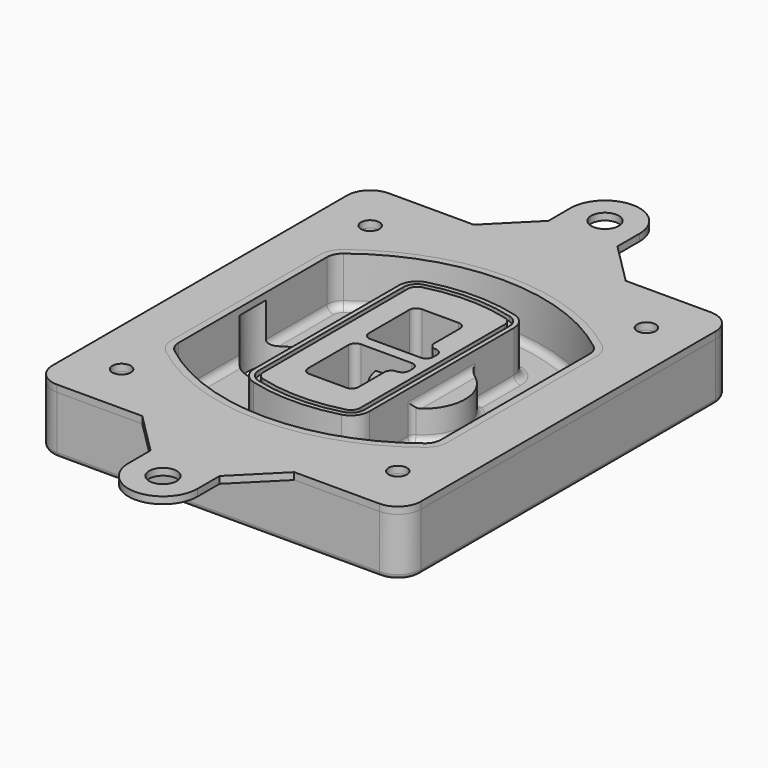
from build123d import *

# Parameters (mm, degrees)
F0_R      = 4
F1_DEPTH  = 25
F2_DEPTH  = 3
F3_DEPTH  = 18
F5_DEPTH  = 21
F6_DEPTH  = 2
F8_DEPTH  = 20
F9_DEPTH  = 16
F10_DEPTH = 25
F7_R      = 6
F7_R_2    = 4
F11_DEPTH = 6
F13_DEPTH = 9
F14_R     = 3
F15_R     = 2
F16_R     = 6
F16_R_2   = 4
F17_DEPTH = 3


with BuildPart() as f1:
    # F0 (on Top) → F1 (new body)
    with BuildSketch(Plane.XY):
        with BuildLine():
            ThreePointArc((-80, -80), (-77.0710678119, -87.0710678119), (-70, -90))
            Line((-70, -90), (70, -90))
            ThreePointArc((70, -90), (77.0710678119, -87.0710678119), (80, -80))
            Line((80, -80), (80, 80))
            ThreePointArc((80, 80), (77.0710678119, 87.0710678119), (70, 90))
            Line((70, 90), (-70, 90))
            ThreePointArc((-70, 90), (-77.0710678119, 87.0710678119), (-80, 80))
            Line((-80, 80), (-80, -80))
        make_face()
        with Locations((-60, -67.5)):
            Circle(F0_R, mode=Mode.SUBTRACT)
        with Locations((60, -67.5)):
            Circle(F0_R, mode=Mode.SUBTRACT)
        with Locations((-60, 67.5)):
            Circle(F0_R, mode=Mode.SUBTRACT)
        with BuildLine():
            ThreePointArc((-64, 40.2934422872), (-62.5820384798, 46.4328484224), (-58.6153846154, 51.3286200352))
            ThreePointArc((-58.6153846154, 51.3286200352), (0, 71.5), (58.6153846154, 51.3286200352))
            ThreePointArc((58.6153846154, 51.3286200352), (62.5820384798, 46.4328484224), (64, 40.2934422872))
            Line((64, 40.2934422872), (64, -40.2934422872))
            ThreePointArc((64, -40.2934422872), (62.5820384798, -46.4328484224), (58.6153846154, -51.3286200352))
            ThreePointArc((58.6153846154, -51.3286200352), (0, -71.5), (-58.6153846154, -51.3286200352))
            ThreePointArc((-58.6153846154, -51.3286200352), (-62.5820384798, -46.4328484224), (-64, -40.2934422872))
            Line((-64, -40.2934422872), (-64, 40.2934422872))
        make_face(mode=Mode.SUBTRACT)
        with Locations((60, 67.5)):
            Circle(F0_R, mode=Mode.SUBTRACT)
        with BuildLine():
            ThreePointArc((58.6153846154, 51.3286200352), (0, 71.5), (-58.6153846154, 51.3286200352))
            ThreePointArc((-58.6153846154, 51.3286200352), (-62.5820384798, 46.4328484224), (-64, 40.2934422872))
            Line((-64, 40.2934422872), (-64, -40.2934422872))
            ThreePointArc((-64, -40.2934422872), (-62.5820384798, -46.4328484224), (-58.6153846154, -51.3286200352))
            ThreePointArc((-58.6153846154, -51.3286200352), (0, -71.5), (58.6153846154, -51.3286200352))
            ThreePointArc((58.6153846154, -51.3286200352), (62.5820384798, -46.4328484224), (64, -40.2934422872))
            Line((64, -40.2934422872), (64, 40.2934422872))
            ThreePointArc((64, 40.2934422872), (62.5820384798, 46.4328484224), (58.6153846154, 51.3286200352))
        make_face()
        with BuildLine():
            Line((-60, -40.2934422872), (-60, 40.2934422872))
            ThreePointArc((-60, 40.2934422872), (-58.9871703427, 44.6787323838), (-56.1538461538, 48.1757121072))
            ThreePointArc((-56.1538461538, 48.1757121072), (0, 67.5), (56.1538461538, 48.1757121072))
            ThreePointArc((56.1538461538, 48.1757121072), (58.9871703427, 44.6787323838), (60, 40.2934422872))
            Line((60, 40.2934422872), (60, -40.2934422872))
            ThreePointArc((60, -40.2934422872), (58.9871703427, -44.6787323838), (56.1538461538, -48.1757121072))
            ThreePointArc((56.1538461538, -48.1757121072), (0, -67.5), (-56.1538461538, -48.1757121072))
            ThreePointArc((-56.1538461538, -48.1757121072), (-58.9871703427, -44.6787323838), (-60, -40.2934422872))
        make_face(mode=Mode.SUBTRACT)
        with BuildLine():
            ThreePointArc((-56.1538461538, 48.1757121072), (-58.9871703427, 44.6787323838), (-60, 40.2934422872))
            Line((-60, 40.2934422872), (-60, -40.2934422872))
            ThreePointArc((-60, -40.2934422872), (-58.9871703427, -44.6787323838), (-56.1538461538, -48.1757121072))
            ThreePointArc((-56.1538461538, -48.1757121072), (0, -67.5), (56.1538461538, -48.1757121072))
            ThreePointArc((56.1538461538, -48.1757121072), (58.9871703427, -44.6787323838), (60, -40.2934422872))
            Line((60, -40.2934422872), (60, 40.2934422872))
            ThreePointArc((60, 40.2934422872), (58.9871703427, 44.6787323838), (56.1538461538, 48.1757121072))
            ThreePointArc((56.1538461538, 48.1757121072), (0, 67.5), (-56.1538461538, 48.1757121072))
        make_face()
        with BuildLine():
            ThreePointArc((54.3076923077, 45.8110311612), (56.2910192399, 43.3631453548), (57, 40.2934422872))
            Line((57, 40.2934422872), (57, -40.2934422872))
            ThreePointArc((57, -40.2934422872), (56.2910192399, -43.3631453548), (54.3076923077, -45.8110311612))
            ThreePointArc((54.3076923077, -45.8110311612), (0, -64.5), (-54.3076923077, -45.8110311612))
            ThreePointArc((-54.3076923077, -45.8110311612), (-56.2910192399, -43.3631453548), (-57, -40.2934422872))
            Line((-57, -40.2934422872), (-57, 40.2934422872))
            ThreePointArc((-57, 40.2934422872), (-56.2910192399, 43.3631453548), (-54.3076923077, 45.8110311612))
            ThreePointArc((-54.3076923077, 45.8110311612), (0, 64.5), (54.3076923077, 45.8110311612))
        make_face(mode=Mode.SUBTRACT)
        with BuildLine():
            Line((57, -40.2934422872), (57, 40.2934422872))
            ThreePointArc((57, 40.2934422872), (56.2910192399, 43.3631453548), (54.3076923077, 45.8110311612))
            ThreePointArc((54.3076923077, 45.8110311612), (0, 64.5), (-54.3076923077, 45.8110311612))
            ThreePointArc((-54.3076923077, 45.8110311612), (-56.2910192399, 43.3631453548), (-57, 40.2934422872))
            Line((-57, 40.2934422872), (-57, -40.2934422872))
            ThreePointArc((-57, -40.2934422872), (-56.2910192399, -43.3631453548), (-54.3076923077, -45.8110311612))
            ThreePointArc((-54.3076923077, -45.8110311612), (0, -64.5), (54.3076923077, -45.8110311612))
            ThreePointArc((54.3076923077, -45.8110311612), (56.2910192399, -43.3631453548), (57, -40.2934422872))
        make_face()
    extrude(amount=-F1_DEPTH)

    # F0 (on Top) → F2 (join)
    with BuildSketch(Plane.XY):
        with BuildLine():
            ThreePointArc((-56.1538461538, 48.1757121072), (-58.9871703427, 44.6787323838), (-60, 40.2934422872))
            Line((-60, 40.2934422872), (-60, -40.2934422872))
            ThreePointArc((-60, -40.2934422872), (-58.9871703427, -44.6787323838), (-56.1538461538, -48.1757121072))
            ThreePointArc((-56.1538461538, -48.1757121072), (0, -67.5), (56.1538461538, -48.1757121072))
            ThreePointArc((56.1538461538, -48.1757121072), (58.9871703427, -44.6787323838), (60, -40.2934422872))
            Line((60, -40.2934422872), (60, 40.2934422872))
            ThreePointArc((60, 40.2934422872), (58.9871703427, 44.6787323838), (56.1538461538, 48.1757121072))
            ThreePointArc((56.1538461538, 48.1757121072), (0, 67.5), (-56.1538461538, 48.1757121072))
        make_face()
        with BuildLine():
            ThreePointArc((54.3076923077, 45.8110311612), (56.2910192399, 43.3631453548), (57, 40.2934422872))
            Line((57, 40.2934422872), (57, -40.2934422872))
            ThreePointArc((57, -40.2934422872), (56.2910192399, -43.3631453548), (54.3076923077, -45.8110311612))
            ThreePointArc((54.3076923077, -45.8110311612), (0, -64.5), (-54.3076923077, -45.8110311612))
            ThreePointArc((-54.3076923077, -45.8110311612), (-56.2910192399, -43.3631453548), (-57, -40.2934422872))
            Line((-57, -40.2934422872), (-57, 40.2934422872))
            ThreePointArc((-57, 40.2934422872), (-56.2910192399, 43.3631453548), (-54.3076923077, 45.8110311612))
            ThreePointArc((-54.3076923077, 45.8110311612), (0, 64.5), (54.3076923077, 45.8110311612))
        make_face(mode=Mode.SUBTRACT)
    extrude(amount=F2_DEPTH)

    # F0 (on Top) → F3 (cut)
    with BuildSketch(Plane.XY):
        with BuildLine():
            Line((57, -40.2934422872), (57, 40.2934422872))
            ThreePointArc((57, 40.2934422872), (56.2910192399, 43.3631453548), (54.3076923077, 45.8110311612))
            ThreePointArc((54.3076923077, 45.8110311612), (0, 64.5), (-54.3076923077, 45.8110311612))
            ThreePointArc((-54.3076923077, 45.8110311612), (-56.2910192399, 43.3631453548), (-57, 40.2934422872))
            Line((-57, 40.2934422872), (-57, -40.2934422872))
            ThreePointArc((-57, -40.2934422872), (-56.2910192399, -43.3631453548), (-54.3076923077, -45.8110311612))
            ThreePointArc((-54.3076923077, -45.8110311612), (0, -64.5), (54.3076923077, -45.8110311612))
            ThreePointArc((54.3076923077, -45.8110311612), (56.2910192399, -43.3631453548), (57, -40.2934422872))
        make_face()
    extrude(amount=-F3_DEPTH, mode=Mode.SUBTRACT)

    # F4 (on face) → F5 (join, through all)
    with BuildSketch(Plane.XY.offset(3)):
        with BuildLine():
            ThreePointArc((-25, -39.2465276821), (-23.3511545998, -44.1109737193), (-19.0842911877, -46.9702398883))
            ThreePointArc((-19.0842911877, -46.9702398883), (0, -49.5), (19.0842911877, -46.9702398883))
            ThreePointArc((19.0842911877, -46.9702398883), (23.3511545998, -44.1109737193), (25, -39.2465276821))
            Line((25, -39.2465276821), (25, 39.2465276821))
            ThreePointArc((25, 39.2465276821), (23.3511545998, 44.1109737193), (19.0842911877, 46.9702398883))
            ThreePointArc((19.0842911877, 46.9702398883), (0, 49.5), (-19.0842911877, 46.9702398883))
            ThreePointArc((-19.0842911877, 46.9702398883), (-23.3511545998, 44.1109737193), (-25, 39.2465276821))
            Line((-25, 39.2465276821), (-25, -39.2465276821))
        make_face()
        with BuildLine():
            ThreePointArc((18.5632183908, 45.0393118368), (21.7633659499, 42.89486221), (23, 39.2465276821))
            Line((23, 39.2465276821), (23, -39.2465276821))
            ThreePointArc((23, -39.2465276821), (21.7633659499, -42.89486221), (18.5632183908, -45.0393118368))
            ThreePointArc((18.5632183908, -45.0393118368), (0, -47.5), (-18.5632183908, -45.0393118368))
            ThreePointArc((-18.5632183908, -45.0393118368), (-21.7633659499, -42.89486221), (-23, -39.2465276821))
            Line((-23, -39.2465276821), (-23, 39.2465276821))
            ThreePointArc((-23, 39.2465276821), (-21.7633659499, 42.89486221), (-18.5632183908, 45.0393118368))
            ThreePointArc((-18.5632183908, 45.0393118368), (0, 47.5), (18.5632183908, 45.0393118368))
        make_face(mode=Mode.SUBTRACT)
        with BuildLine():
            Line((23, -39.2465276821), (23, 39.2465276821))
            ThreePointArc((23, 39.2465276821), (21.7633659499, 42.89486221), (18.5632183908, 45.0393118368))
            ThreePointArc((18.5632183908, 45.0393118368), (0, 47.5), (-18.5632183908, 45.0393118368))
            ThreePointArc((-18.5632183908, 45.0393118368), (-21.7633659499, 42.89486221), (-23, 39.2465276821))
            Line((-23, 39.2465276821), (-23, -39.2465276821))
            ThreePointArc((-23, -39.2465276821), (-21.7633659499, -42.89486221), (-18.5632183908, -45.0393118368))
            ThreePointArc((-18.5632183908, -45.0393118368), (0, -47.5), (18.5632183908, -45.0393118368))
            ThreePointArc((18.5632183908, -45.0393118368), (21.7633659499, -42.89486221), (23, -39.2465276821))
        make_face()
        with BuildLine():
            ThreePointArc((18.0421455939, 43.1083837852), (20.1755772999, 41.6787507007), (21, 39.2465276821))
            Line((21, 39.2465276821), (21, -39.2465276821))
            ThreePointArc((21, -39.2465276821), (20.1755772999, -41.6787507007), (18.0421455939, -43.1083837852))
            ThreePointArc((18.0421455939, -43.1083837852), (0, -45.5), (-18.0421455939, -43.1083837852))
            ThreePointArc((-18.0421455939, -43.1083837852), (-20.1755772999, -41.6787507007), (-21, -39.2465276821))
            Line((-21, -39.2465276821), (-21, 39.2465276821))
            ThreePointArc((-21, 39.2465276821), (-20.1755772999, 41.6787507007), (-18.0421455939, 43.1083837852))
            ThreePointArc((-18.0421455939, 43.1083837852), (0, 45.5), (18.0421455939, 43.1083837852))
        make_face(mode=Mode.SUBTRACT)
        with BuildLine():
            Line((21, -39.2465276821), (21, 39.2465276821))
            ThreePointArc((21, 39.2465276821), (20.1755772999, 41.6787507007), (18.0421455939, 43.1083837852))
            ThreePointArc((18.0421455939, 43.1083837852), (0, 45.5), (-18.0421455939, 43.1083837852))
            ThreePointArc((-18.0421455939, 43.1083837852), (-20.1755772999, 41.6787507007), (-21, 39.2465276821))
            Line((-21, 39.2465276821), (-21, -39.2465276821))
            ThreePointArc((-21, -39.2465276821), (-20.1755772999, -41.6787507007), (-18.0421455939, -43.1083837852))
            ThreePointArc((-18.0421455939, -43.1083837852), (0, -45.5), (18.0421455939, -43.1083837852))
            ThreePointArc((18.0421455939, -43.1083837852), (20.1755772999, -41.6787507007), (21, -39.2465276821))
        make_face()
        with BuildLine():
            Line((-8, -2.5), (14, -2.5))
            ThreePointArc((14, -2.5), (16.1213203436, -3.3786796564), (17, -5.5))
            Line((17, -5.5), (17, -7.5))
            ThreePointArc((17, -7.5), (16.1213203436, -9.6213203436), (14, -10.5))
            ThreePointArc((14, -10.5), (11.8786796564, -11.3786796564), (11, -13.5))
            Line((11, -13.5), (11, -27.5))
            ThreePointArc((11, -27.5), (10.1213203436, -29.6213203436), (8, -30.5))
            Line((8, -30.5), (-8, -30.5))
            ThreePointArc((-8, -30.5), (-10.1213203436, -29.6213203436), (-11, -27.5))
            Line((-11, -27.5), (-11, -5.5))
            ThreePointArc((-11, -5.5), (-10.1213203436, -3.3786796564), (-8, -2.5))
        make_face(mode=Mode.SUBTRACT)
        with BuildLine():
            ThreePointArc((-8, 2.5), (-10.1213203436, 3.3786796564), (-11, 5.5))
            Line((-11, 5.5), (-11, 27.5))
            ThreePointArc((-11, 27.5), (-10.1213203436, 29.6213203436), (-8, 30.5))
            Line((-8, 30.5), (8, 30.5))
            ThreePointArc((8, 30.5), (10.1213203436, 29.6213203436), (11, 27.5))
            Line((11, 27.5), (11, 13.5))
            ThreePointArc((11, 13.5), (11.8786796564, 11.3786796564), (14, 10.5))
            ThreePointArc((14, 10.5), (16.1213203436, 9.6213203436), (17, 7.5))
            Line((17, 7.5), (17, 5.5))
            ThreePointArc((17, 5.5), (16.1213203436, 3.3786796564), (14, 2.5))
            Line((14, 2.5), (-8, 2.5))
        make_face(mode=Mode.SUBTRACT)
    extrude(amount=-F5_DEPTH)

    # F4 (on face) → F6 (cut)
    with BuildSketch(Plane.XY.offset(3)):
        with BuildLine():
            Line((23, -39.2465276821), (23, 39.2465276821))
            ThreePointArc((23, 39.2465276821), (21.7633659499, 42.89486221), (18.5632183908, 45.0393118368))
            ThreePointArc((18.5632183908, 45.0393118368), (0, 47.5), (-18.5632183908, 45.0393118368))
            ThreePointArc((-18.5632183908, 45.0393118368), (-21.7633659499, 42.89486221), (-23, 39.2465276821))
            Line((-23, 39.2465276821), (-23, -39.2465276821))
            ThreePointArc((-23, -39.2465276821), (-21.7633659499, -42.89486221), (-18.5632183908, -45.0393118368))
            ThreePointArc((-18.5632183908, -45.0393118368), (0, -47.5), (18.5632183908, -45.0393118368))
            ThreePointArc((18.5632183908, -45.0393118368), (21.7633659499, -42.89486221), (23, -39.2465276821))
        make_face()
        with BuildLine():
            ThreePointArc((18.0421455939, 43.1083837852), (20.1755772999, 41.6787507007), (21, 39.2465276821))
            Line((21, 39.2465276821), (21, -39.2465276821))
            ThreePointArc((21, -39.2465276821), (20.1755772999, -41.6787507007), (18.0421455939, -43.1083837852))
            ThreePointArc((18.0421455939, -43.1083837852), (0, -45.5), (-18.0421455939, -43.1083837852))
            ThreePointArc((-18.0421455939, -43.1083837852), (-20.1755772999, -41.6787507007), (-21, -39.2465276821))
            Line((-21, -39.2465276821), (-21, 39.2465276821))
            ThreePointArc((-21, 39.2465276821), (-20.1755772999, 41.6787507007), (-18.0421455939, 43.1083837852))
            ThreePointArc((-18.0421455939, 43.1083837852), (0, 45.5), (18.0421455939, 43.1083837852))
        make_face(mode=Mode.SUBTRACT)
    extrude(amount=-F6_DEPTH, mode=Mode.SUBTRACT)

    # F7 (on face) → F8 (join)
    with BuildSketch(Plane(origin=(0, 0, -25), x_dir=(1, 0, 0), z_dir=(0, 0, -1))):
        with BuildLine():
            ThreePointArc((3.28842436, 0), (16.7567035675, 13.4682792075), (30.224982775, 0))
            Line((30.224982775, 0), (35.224982775, 0))
            ThreePointArc((35.224982775, 0), (16.7567035675, 18.4682792075), (-1.71157564, 0))
            Line((-1.71157564, 0), (3.28842436, 0))
        make_face()
        with BuildLine():
            Line((3.28842436, 0), (30.224982775, 0))
            ThreePointArc((30.224982775, 0), (16.7567035675, 13.4682792075), (3.28842436, 0))
        make_face()
        with BuildLine():
            ThreePointArc((3.28842436, 0), (16.7567035675, -13.4682792075), (30.224982775, 0))
            Line((30.224982775, 0), (3.28842436, 0))
        make_face()
        with BuildLine():
            Line((35.224982775, 0), (30.224982775, 0))
            ThreePointArc((30.224982775, 0), (16.7567035675, -13.4682792075), (3.28842436, 0))
            Line((3.28842436, 0), (-1.71157564, 0))
            ThreePointArc((-1.71157564, 0), (16.7567035675, -18.4682792075), (35.224982775, 0))
        make_face()
    extrude(amount=-F8_DEPTH)

    # F7 (on face) → F9 (cut)
    with BuildSketch(Plane(origin=(0, 0, -25), x_dir=(1, 0, 0), z_dir=(0, 0, -1))):
        with BuildLine():
            Line((3.28842436, 0), (30.224982775, 0))
            ThreePointArc((30.224982775, 0), (16.7567035675, 13.4682792075), (3.28842436, 0))
        make_face()
        with BuildLine():
            ThreePointArc((3.28842436, 0), (16.7567035675, -13.4682792075), (30.224982775, 0))
            Line((30.224982775, 0), (3.28842436, 0))
        make_face()
    extrude(amount=-F9_DEPTH, mode=Mode.SUBTRACT)

    # F7 (on face) → F10 (cut)
    with BuildSketch(Plane(origin=(0, 0, -25), x_dir=(1, 0, 0), z_dir=(0, 0, -1))):
        with BuildLine():
            Line((-59.0318229325, 0), (-32.0952645175, 0))
            ThreePointArc((-32.0952645175, 0), (-45.563543725, 13.4682792075), (-59.0318229325, 0))
        make_face()
        with BuildLine():
            ThreePointArc((-59.0318229325, 0), (-45.563543725, -13.4682792075), (-32.0952645175, 0))
            Line((-32.0952645175, 0), (-59.0318229325, 0))
        make_face()
    extrude(amount=-F10_DEPTH, mode=Mode.SUBTRACT)

    # F7 (on face) → F11 (cut)
    with BuildSketch(Plane(origin=(0, 0, -25), x_dir=(1, 0, 0), z_dir=(0, 0, -1))):
        with Locations((60, -67.5)):
            Circle(F7_R)
        with Locations((60, -67.5)):
            Circle(F7_R_2, mode=Mode.SUBTRACT)
        with Locations((-60, -67.5)):
            Circle(F7_R)
        with Locations((-60, -67.5)):
            Circle(F7_R_2, mode=Mode.SUBTRACT)
        with Locations((-60, 67.5)):
            Circle(F7_R)
        with Locations((-60, 67.5)):
            Circle(F7_R_2, mode=Mode.SUBTRACT)
        with Locations((60, 67.5)):
            Circle(F7_R)
        with Locations((60, 67.5)):
            Circle(F7_R_2, mode=Mode.SUBTRACT)
    extrude(amount=-F11_DEPTH, mode=Mode.SUBTRACT)

    # F12 (on face) → F13 (cut, through all)
    with BuildSketch(Plane(origin=(0, 0, -9), x_dir=(1, 0, 0), z_dir=(0, 0, -1))):
        with BuildLine():
            Line((11, 13.5), (11, 17.5481537753))
            ThreePointArc((11, 17.5481537753), (2.5696536419, 11.8239143813), (-1.5415842455, 2.5))
            Line((-1.5415842455, 2.5), (3.5224848595, 2.5))
            ThreePointArc((3.5224848595, 2.5), (6.1857188154, 8.3455872281), (11.2536447004, 12.2927168648))
            ThreePointArc((11.2536447004, 12.2927168648), (11.0640958889, 12.8831798879), (11, 13.5))
        make_face()
        with BuildLine():
            ThreePointArc((11.2536447004, -12.2927168648), (6.1857188154, -8.3455872281), (3.5224848595, -2.5))
            Line((3.5224848595, -2.5), (-1.5415842455, -2.5))
            ThreePointArc((-1.5415842455, -2.5), (2.5696536419, -11.8239143813), (11, -17.5481537753))
            Line((11, -17.5481537753), (11, -13.5))
            ThreePointArc((11, -13.5), (11.0640958889, -12.8831798879), (11.2536447004, -12.2927168648))
        make_face()
        with BuildLine():
            ThreePointArc((11.2536447004, 12.2927168648), (6.1857188154, 8.3455872281), (3.5224848595, 2.5))
            Line((3.5224848595, 2.5), (14, 2.5))
            ThreePointArc((14, 2.5), (16.1213203436, 3.3786796564), (17, 5.5))
            Line((17, 5.5), (17, 7.5))
            ThreePointArc((17, 7.5), (16.1213203436, 9.6213203436), (14, 10.5))
            ThreePointArc((14, 10.5), (12.3601599782, 10.9878446101), (11.2536447004, 12.2927168648))
        make_face()
        with BuildLine():
            Line((14, -2.5), (3.5224848595, -2.5))
            ThreePointArc((3.5224848595, -2.5), (6.1857188154, -8.3455872281), (11.2536447004, -12.2927168648))
            ThreePointArc((11.2536447004, -12.2927168648), (12.3601599782, -10.9878446101), (14, -10.5))
            ThreePointArc((14, -10.5), (16.1213203436, -9.6213203436), (17, -7.5))
            Line((17, -7.5), (17, -5.5))
            ThreePointArc((17, -5.5), (16.1213203436, -3.3786796564), (14, -2.5))
        make_face()
    extrude(amount=F13_DEPTH, mode=Mode.SUBTRACT)

    # F14
    f14_edges = [f1.edges().sort_by_distance(p)[0] for p in [
        (-57, -23.703476, -18),
        (-57, 23.703476, -18),
        (25, 0, -5),
        (25, 16.526506, -11.5),
        (25, -16.526506, -11.5),
        (25, -27.886517, -18),
        (35.224983, 0, -18),
    ]]
    fillet(f14_edges, radius=F14_R)

    # F15
    f15_edges = [f1.edges().sort_by_distance(p)[0] for p in [
        (0, -90, -25),
    ]]
    fillet(f15_edges, radius=F15_R)


with BuildPart() as f17:
    # F16 (on face) → F17 (new body, through all)
    with BuildSketch(Plane.XY):
        with BuildLine():
            Line((-33, 90), (33, 90))
            Line((33, 90), (15, 108))
            Line((15, 108), (15, 120))
            ThreePointArc((15, 120), (0, 135), (-15, 120))
            Line((-15, 120), (-15, 108))
            Line((-15, 108), (-33, 90))
        make_face()
        with Locations((0, 120)):
            Circle(F16_R, mode=Mode.SUBTRACT)
        with BuildLine():
            Line((15, -108), (33, -90))
            Line((33, -90), (-33, -90))
            Line((-33, -90), (-15, -108))
            Line((-15, -108), (-15, -120))
            ThreePointArc((-15, -120), (0, -135), (15, -120))
            Line((15, -120), (15, -108))
        make_face()
        with Locations((0, -120)):
            Circle(F16_R, mode=Mode.SUBTRACT)
        with BuildLine():
            ThreePointArc((80, 80), (77.0710678119, 87.0710678119), (70, 90))
            Line((70, 90), (33, 90))
            Line((33, 90), (-33, 90))
            Line((-33, 90), (-70, 90))
            ThreePointArc((-70, 90), (-77.0710678119, 87.0710678119), (-80, 80))
            Line((-80, 80), (-80, -80))
            ThreePointArc((-80, -80), (-77.0710678119, -87.0710678119), (-70, -90))
            Line((-70, -90), (-33, -90))
            Line((-33, -90), (33, -90))
            Line((33, -90), (70, -90))
            ThreePointArc((70, -90), (77.0710678119, -87.0710678119), (80, -80))
            Line((80, -80), (80, 80))
        make_face()
        with Locations((-60, -67.5)):
            Circle(F16_R_2, mode=Mode.SUBTRACT)
        with BuildLine():
            Line((60, 40.2934422872), (60, -40.2934422872))
            ThreePointArc((60, -40.2934422872), (58.9871703427, -44.6787323838), (56.1538461538, -48.1757121072))
            ThreePointArc((56.1538461538, -48.1757121072), (0, -67.5), (-56.1538461538, -48.1757121072))
            ThreePointArc((-56.1538461538, -48.1757121072), (-58.9871703427, -44.6787323838), (-60, -40.2934422872))
            Line((-60, -40.2934422872), (-60, 40.2934422872))
            ThreePointArc((-60, 40.2934422872), (-58.9871703427, 44.6787323838), (-56.1538461538, 48.1757121072))
            ThreePointArc((-56.1538461538, 48.1757121072), (0, 67.5), (56.1538461538, 48.1757121072))
            ThreePointArc((56.1538461538, 48.1757121072), (58.9871703427, 44.6787323838), (60, 40.2934422872))
        make_face(mode=Mode.SUBTRACT)
        with Locations((60, -67.5)):
            Circle(F16_R_2, mode=Mode.SUBTRACT)
        with Locations((-60, 67.5)):
            Circle(F16_R_2, mode=Mode.SUBTRACT)
        with Locations((60, 67.5)):
            Circle(F16_R_2, mode=Mode.SUBTRACT)
    extrude(amount=F17_DEPTH)


solid = Compound([f1.part, f17.part])
